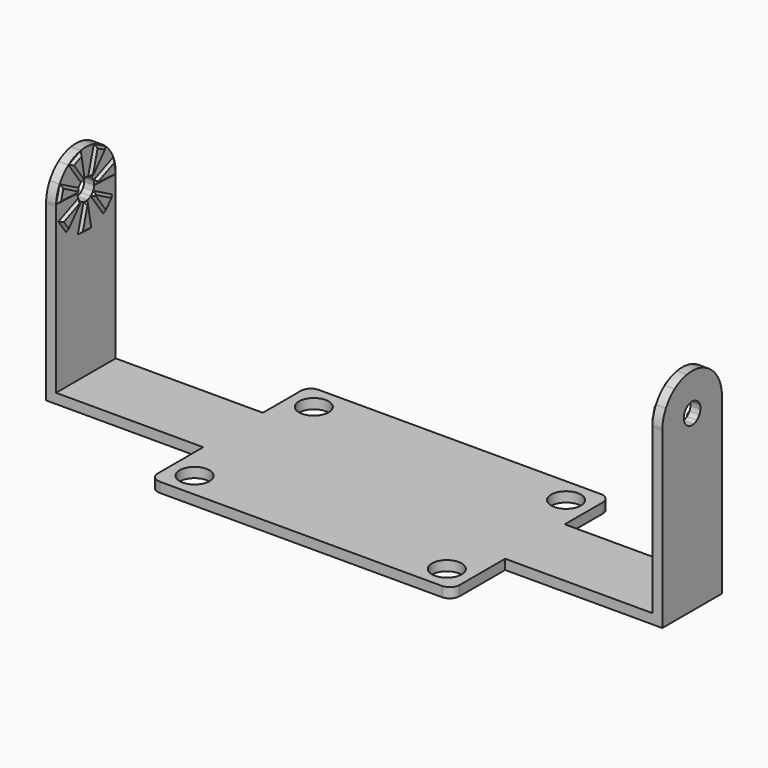
from build123d import *

# Parameters (mm, degrees)
F0_R                     = 3
F1_DEPTH                 = 2
F3_W                     = 29.6193578921
F3_H                     = 8.8474444038
F3_H_2                   = 6.1525555962
F4_DEPTH                 = 2
F6_DEPTH                 = 2
F7_DEPTH                 = 2
F8_DEPTH                 = 0.5
DRAFT_F8_DRAFTED_ANGLE   = 45
DRAFT_F8_2_DRAFTED_ANGLE = 45
DRAFT_F8_3_DRAFTED_ANGLE = 45
DRAFT_F8_4_DRAFTED_ANGLE = 45
DRAFT_F8_5_DRAFTED_ANGLE = 45
DRAFT_F8_6_DRAFTED_ANGLE = 45
DRAFT_F8_7_DRAFTED_ANGLE = 45


# Not quite as in the source:
# - an extrude with a draft is written as a straight extrude whose walls are then drafted
# - a feature names something its author has since deleted; it is built from what else it names


with BuildPart() as f1:
    # F0 (on Top) → F1 (new body)
    with BuildSketch(Plane.XY):
        with BuildLine():
            Line((0, 20.4223022205), (-28.3806421079, 20.4223022205))
            ThreePointArc((-28.3806421079, 20.4223022205), (-29.7948556703, 19.8365157828), (-30.3806421079, 18.4223022205))
            Line((-30.3806421079, 18.4223022205), (-30.3806421079, -17.5776977795))
            ThreePointArc((-30.3806421079, -17.5776977795), (-29.7948556703, -18.9919113419), (-28.3806421079, -19.5776977795))
            Line((-28.3806421079, -19.5776977795), (0, -19.5776977795))
            Line((0, -19.5776977795), (0, 20.4223022205))
        make_face()
        with Locations((-25.3806421079, -14.5776977795)):
            Circle(F0_R, mode=Mode.SUBTRACT)
        with Locations((-25.3806421079, 15.4223022205)):
            Circle(F0_R, mode=Mode.SUBTRACT)
    extrude(amount=F1_DEPTH)

    # F3 (on face) → F4 (join)
    with BuildSketch(Plane.XY.offset(2)):
        with Locations((-45.190321054, 4.4237222019)):
            Rectangle(F3_W, F3_H)
        with Locations((-45.190321054, -3.0762777981)):
            Rectangle(F3_W, F3_H_2)
    extrude(amount=-F4_DEPTH)

    # F5 (on face) → F6 (join)
    with BuildSketch(Plane(origin=(-60, 0, 0), x_dir=(0, -1, 0), z_dir=(-1, 0, 0))):
        with BuildLine():
            ThreePointArc((5.5633466733, 32.0864426173), (6.0037777081, 33.5139190004), (6.1525555962, 35.0003689528))
            ThreePointArc((6.1525555962, 35.0003689528), (6.1502334534, 35.1869882142), (6.1432684632, 35.373491914))
            Line((6.1432684632, 35.373491914), (5.5633466733, 32.0864426173))
        make_face()
        with BuildLine():
            Line((6.1525555962, 2), (6.1525555962, 35.0003689528))
            ThreePointArc((6.1525555962, 35.0003689528), (6.0037777081, 33.5139190004), (5.5633466733, 32.0864426173))
            ThreePointArc((5.5633466733, 32.0864426173), (4.7416691029, 30.6217051494), (3.6146579553, 29.3765321684))
            ThreePointArc((3.6146579553, 29.3765321684), (2.2388262755, 28.4133618467), (0.6831640089, 27.7804915664))
            ThreePointArc((0.6831640089, 27.7804915664), (-0.9743214426, 27.5096560858), (-2.6505168374, 27.6144362268))
            ThreePointArc((-2.6505168374, 27.6144362268), (-4.2613707393, 28.0895778756), (-5.7261082072, 28.9112554461))
            ThreePointArc((-5.7261082072, 28.9112554461), (-6.9712811882, 30.0382665936), (-7.9344515098, 31.4140982734))
            ThreePointArc((-7.9344515098, 31.4140982734), (-8.5673217902, 32.96976054), (-8.8381572708, 34.6272459916))
            ThreePointArc((-8.8381572708, 34.6272459916), (-8.8451176686, 34.8135652721), (-8.8474443948, 35))
            Line((-8.8474444038, 35), (-8.8474444038, 2))
            Line((-8.8474444038, 2), (6.1525555962, 2))
        make_face()
        with BuildLine():
            Line((5.2395627022, 38.5866396321), (6.1432684632, 35.373491914))
            ThreePointArc((6.1432684632, 35.373491914), (5.8724329825, 37.0309773655), (5.2395627022, 38.5866396321))
        make_face()
        with BuildLine():
            Line((0.7499551989, 35.1048433819), (6.1432684632, 35.373491914))
            Line((6.1432684632, 35.373491914), (5.2395627022, 38.5866396321))
            Line((5.2395627022, 38.5866396321), (0.4969175858, 36.004524743))
            ThreePointArc((0.4969175858, 36.004524743), (0.6741212644, 35.5689393083), (0.7499551989, 35.1048433819))
        make_face()
        with BuildLine():
            Line((5.5633466733, 32.0864426173), (6.1432684632, 35.373491914))
            Line((6.1432684632, 35.373491914), (0.7499551989, 35.1048433819))
            ThreePointArc((0.7499551989, 35.1048433819), (0.7519053962, 35.052622346), (0.7525555962, 35.0003689528))
            ThreePointArc((0.7525555962, 35.0003689528), (0.7108977875, 34.5841629661), (0.5875770978, 34.1844695788))
            Line((0.5875770978, 34.1844695788), (5.5633466733, 32.0864426173))
        make_face()
        with BuildLine():
            ThreePointArc((3.6146579553, 29.3765321684), (4.7416691029, 30.6217051494), (5.5633466733, 32.0864426173))
            Line((5.5633466733, 32.0864426173), (3.6146579553, 29.3765321684))
        make_face()
        with BuildLine():
            Line((3.6146579553, 29.3765321684), (5.5633466733, 32.0864426173))
            Line((5.5633466733, 32.0864426173), (0.5875770978, 34.1844695788))
            ThreePointArc((0.5875770978, 34.1844695788), (0.357507378, 33.7743430878), (0.0419442567, 33.4256946531))
            Line((0.0419442567, 33.4256946531), (3.6146579553, 29.3765321684))
        make_face()
        with BuildLine():
            Line((3.0312193995, 41.0894824594), (5.2395627022, 38.5866396321))
            ThreePointArc((5.2395627022, 38.5866396321), (4.2763923806, 39.9624713119), (3.0312193995, 41.0894824594))
        make_face()
        with BuildLine():
            Line((0.4969175858, 36.004524743), (5.2395627022, 38.5866396321))
            Line((5.2395627022, 38.5866396321), (3.0312193995, 41.0894824594))
            Line((3.0312193995, 41.0894824594), (-0.1214185389, 36.7053207346))
            ThreePointArc((-0.1214185389, 36.7053207346), (0.2272298958, 36.3897576133), (0.4969175858, 36.004524743))
        make_face()
        with BuildLine():
            ThreePointArc((0.6831640089, 27.7804915664), (2.2388262755, 28.4133618467), (3.6146579553, 29.3765321684))
            Line((3.6146579553, 29.3765321684), (0.6831640089, 27.7804915664))
        make_face()
        with BuildLine():
            Line((0.6831640089, 27.7804915664), (3.6146579553, 29.3765321684))
            Line((3.6146579553, 29.3765321684), (0.0419442567, 33.4256946531))
            ThreePointArc((0.0419442567, 33.4256946531), (-0.3432886136, 33.1560069631), (-0.7788740483, 32.9788032846))
            Line((-0.7788740483, 32.9788032846), (0.6831640089, 27.7804915664))
        make_face()
        with BuildLine():
            Line((-0.0443719702, 42.3863016787), (3.0312193995, 41.0894824594))
            ThreePointArc((3.0312193995, 41.0894824594), (1.5664819316, 41.9111600299), (-0.0443719702, 42.3863016787))
        make_face()
        with BuildLine():
            Line((-0.1214185389, 36.7053207346), (3.0312193995, 41.0894824594))
            Line((3.0312193995, 41.0894824594), (-0.0443719702, 42.3863016787))
            Line((-0.0443719702, 42.3863016787), (-0.9825841224, 37.068430116))
            ThreePointArc((-0.9825841224, 37.068430116), (-0.5315450299, 36.9353904543), (-0.1214185389, 36.7053207346))
        make_face()
        with BuildLine():
            ThreePointArc((-2.6505168374, 27.6144362268), (-0.9743214426, 27.5096560858), (0.6831640089, 27.7804915664))
            Line((0.6831640089, 27.7804915664), (-2.6505168374, 27.6144362268))
        make_face()
        with BuildLine():
            Line((-2.6505168374, 27.6144362268), (0.6831640089, 27.7804915664))
            Line((0.6831640089, 27.7804915664), (-0.7788740483, 32.9788032846))
            ThreePointArc((-0.7788740483, 32.9788032846), (-1.2429699747, 32.90296935), (-1.7123046852, 32.9323077895))
            Line((-1.7123046852, 32.9323077895), (-2.6505168374, 27.6144362268))
        make_face()
        with BuildLine():
            ThreePointArc((-8.258235481, 37.9142952882), (-8.6987030755, 36.4866380877), (-8.8474443948, 35))
            ThreePointArc((-8.8474443948, 35), (-8.8451176686, 34.8135652721), (-8.8381572708, 34.6272459916))
            Line((-8.8381572708, 34.6272459916), (-8.258235481, 37.9142952882))
        make_face()
        with BuildLine():
            Line((-3.3780528165, 42.2202463391), (-0.0443719702, 42.3863016787))
            ThreePointArc((-0.0443719702, 42.3863016787), (-1.720567365, 42.4910818198), (-3.3780528165, 42.2202463391))
        make_face()
        with BuildLine():
            Line((-0.9825841224, 37.068430116), (-0.0443719702, 42.3863016787))
            Line((-0.0443719702, 42.3863016787), (-3.3780528165, 42.2202463391))
            Line((-3.3780528165, 42.2202463391), (-1.9160147594, 37.0219346209))
            ThreePointArc((-1.9160147594, 37.0219346209), (-1.451918833, 37.0977685555), (-0.9825841224, 37.068430116))
        make_face()
        with BuildLine():
            Line((-8.258235481, 37.9142952882), (-3.2824659054, 35.8162683267))
            ThreePointArc((-3.2824659054, 35.8162683267), (-3.0523961857, 36.2263948177), (-2.7368330644, 36.5750432524))
            Line((-2.7368330644, 36.5750432524), (-6.309546763, 40.6242057372))
            Line((-6.309546763, 40.6242057372), (-8.258235481, 37.9142952882))
        make_face()
        with BuildLine():
            ThreePointArc((-3.4448440066, 34.8958945236), (-3.4155055671, 35.3652292342), (-3.2824659054, 35.8162683267))
            Line((-3.2824659054, 35.8162683267), (-8.258235481, 37.9142952882))
            Line((-8.258235481, 37.9142952882), (-8.8381572708, 34.6272459916))
            Line((-8.8381572708, 34.6272459916), (-3.4448440066, 34.8958945236))
        make_face()
        with BuildLine():
            Line((-6.309546763, 40.6242057372), (-2.7368330644, 36.5750432524))
            ThreePointArc((-2.7368330644, 36.5750432524), (-2.351600194, 36.8447309424), (-1.9160147594, 37.0219346209))
            Line((-1.9160147594, 37.0219346209), (-3.3780528165, 42.2202463391))
            Line((-3.3780528165, 42.2202463391), (-6.309546763, 40.6242057372))
        make_face()
        with BuildLine():
            Line((-2.6505168374, 27.6144362268), (-1.7123046852, 32.9323077895))
            ThreePointArc((-1.7123046852, 32.9323077895), (-2.1633437778, 33.0653474512), (-2.5734702688, 33.2954171709))
            Line((-2.5734702688, 33.2954171709), (-5.7261082072, 28.9112554461))
            Line((-5.7261082072, 28.9112554461), (-2.6505168374, 27.6144362268))
        make_face()
        with BuildLine():
            Line((-5.7261082072, 28.9112554461), (-2.5734702688, 33.2954171709))
            ThreePointArc((-2.5734702688, 33.2954171709), (-2.9221187035, 33.6109802922), (-3.1918063935, 33.9962131625))
            Line((-3.1918063935, 33.9962131625), (-7.9344515098, 31.4140982734))
            Line((-7.9344515098, 31.4140982734), (-5.7261082072, 28.9112554461))
        make_face()
        with BuildLine():
            Line((-7.9344515098, 31.4140982734), (-3.1918063935, 33.9962131625))
            ThreePointArc((-3.1918063935, 33.9962131625), (-3.369010072, 34.4317985972), (-3.4448440066, 34.8958945236))
            Line((-3.4448440066, 34.8958945236), (-8.8381572708, 34.6272459916))
            Line((-8.8381572708, 34.6272459916), (-7.9344515098, 31.4140982734))
        make_face()
        with BuildLine():
            ThreePointArc((-5.7261082072, 28.9112554461), (-4.2613707393, 28.0895778756), (-2.6505168374, 27.6144362268))
            Line((-2.6505168374, 27.6144362268), (-5.7261082072, 28.9112554461))
        make_face()
        with BuildLine():
            ThreePointArc((-6.309546763, 40.6242057372), (-7.4365579105, 39.3790327561), (-8.258235481, 37.9142952882))
            Line((-8.258235481, 37.9142952882), (-6.309546763, 40.6242057372))
        make_face()
        with BuildLine():
            Line((-7.9344515098, 31.4140982734), (-8.8381572708, 34.6272459916))
            ThreePointArc((-8.8381572708, 34.6272459916), (-8.5673217902, 32.96976054), (-7.9344515098, 31.4140982734))
        make_face()
        with BuildLine():
            Line((-6.309546763, 40.6242057372), (-3.3780528165, 42.2202463391))
            ThreePointArc((-3.3780528165, 42.2202463391), (-4.9337150832, 41.5873760588), (-6.309546763, 40.6242057372))
        make_face()
        with BuildLine():
            ThreePointArc((-7.9344515098, 31.4140982734), (-6.9712811882, 30.0382665936), (-5.7261082072, 28.9112554461))
            Line((-5.7261082072, 28.9112554461), (-7.9344515098, 31.4140982734))
        make_face()
    extrude(amount=F6_DEPTH)

    # F7 (add): a face of the model
    f7_faces = [f1.faces().sort_by_distance(p)[0] for p in [
        (-60, 1.3474444038, 1),
    ]]
    extrude(f7_faces, amount=F7_DEPTH)


with BuildPart() as f8_drafted:
    # F5 (on face) → F8 (new body)
    with BuildSketch(Plane(origin=(-60, 0, 0), x_dir=(0, -1, 0), z_dir=(-1, 0, 0))):
        with BuildLine():
            Line((3.6146579553, 29.3765321684), (5.5633466733, 32.0864426173))
            Line((5.5633466733, 32.0864426173), (0.5875770978, 34.1844695788))
            ThreePointArc((0.5875770978, 34.1844695788), (0.357507378, 33.7743430878), (0.0419442567, 33.4256946531))
            Line((0.0419442567, 33.4256946531), (3.6146579553, 29.3765321684))
        make_face()
    extrude(amount=-F8_DEPTH)

    # draft_F8_drafted
    draft_f8_drafted_walls = [f8_drafted.faces().sort_by_distance(p)[0] for p in [
        (-59.6666666667, -0.357507378, 33.7743430878),
        (-59.6666666667, -1.828301106, 31.4011134107),
        (-59.6666666667, -4.5890023143, 30.7314873928),
        (-59.6666666667, -3.0754618855, 33.1354560981),
    ]]
    draft(draft_f8_drafted_walls, neutral_plane=Plane(origin=(-60, 0, 0), x_dir=(0, -1, 0), z_dir=(1, 0, 0)), angle=DRAFT_F8_DRAFTED_ANGLE)


with BuildPart() as f1_1:
    add(f1.part)

    # join_F8_drafted: union F8_drafted
    add(f8_drafted.part)


with BuildPart() as f8_2_drafted:
    # F5 (on face) → F8, piece 2 (new body)
    with BuildSketch(Plane(origin=(-60, 0, 0), x_dir=(0, -1, 0), z_dir=(-1, 0, 0))):
        with BuildLine():
            Line((0.7499551989, 35.1048433819), (6.1432684632, 35.373491914))
            Line((6.1432684632, 35.373491914), (5.2395627022, 38.5866396321))
            Line((5.2395627022, 38.5866396321), (0.4969175858, 36.004524743))
            ThreePointArc((0.4969175858, 36.004524743), (0.6741212644, 35.5689393083), (0.7499551989, 35.1048433819))
        make_face()
    extrude(amount=-F8_DEPTH)

    # draft_F8_2_drafted
    draft_f8_2_drafted_walls = [f8_2_drafted.faces().sort_by_distance(p)[0] for p in [
        (-59.6666666667, -0.6741212644, 35.5689393083),
        (-59.6666666667, -3.446611831, 35.2391676479),
        (-59.6666666667, -5.6914155827, 36.980065773),
        (-59.6666666667, -2.868240144, 37.2955821875),
    ]]
    draft(draft_f8_2_drafted_walls, neutral_plane=Plane(origin=(-60, 0, 0), x_dir=(0, -1, 0), z_dir=(1, 0, 0)), angle=DRAFT_F8_2_DRAFTED_ANGLE)


with BuildPart() as f1_2:
    add(f1_1.part)

    # join_F8_2_drafted: union F8_2_drafted
    add(f8_2_drafted.part)


with BuildPart() as f8_3_drafted:
    # F5 (on face) → F8, piece 3 (new body)
    with BuildSketch(Plane(origin=(-60, 0, 0), x_dir=(0, -1, 0), z_dir=(-1, 0, 0))):
        with BuildLine():
            Line((-0.1214185389, 36.7053207346), (3.0312193995, 41.0894824594))
            Line((3.0312193995, 41.0894824594), (-0.0443719702, 42.3863016787))
            Line((-0.0443719702, 42.3863016787), (-0.9825841224, 37.068430116))
            ThreePointArc((-0.9825841224, 37.068430116), (-0.5315450299, 36.9353904543), (-0.1214185389, 36.7053207346))
        make_face()
    extrude(amount=-F8_DEPTH)

    # draft_F8_3_drafted
    draft_f8_3_drafted_walls = [f8_3_drafted.faces().sort_by_distance(p)[0] for p in [
        (-59.6666666667, -1.4549004303, 38.897401597),
        (-59.6666666667, -1.4934237146, 41.7378920691),
        (-59.6666666667, 0.5134780463, 39.7273658974),
        (-59.6666666667, 0.5315450299, 36.9353904543),
    ]]
    draft(draft_f8_3_drafted_walls, neutral_plane=Plane(origin=(-60, 0, 0), x_dir=(0, -1, 0), z_dir=(1, 0, 0)), angle=DRAFT_F8_3_DRAFTED_ANGLE)


with BuildPart() as f1_3:
    add(f1_2.part)

    # join_F8_3_drafted: union F8_3_drafted
    add(f8_3_drafted.part)


with BuildPart() as f8_4_drafted:
    # F5 (on face) → F8, piece 4 (new body)
    with BuildSketch(Plane(origin=(-60, 0, 0), x_dir=(0, -1, 0), z_dir=(-1, 0, 0))):
        with BuildLine():
            Line((-6.309546763, 40.6242057372), (-2.7368330644, 36.5750432524))
            ThreePointArc((-2.7368330644, 36.5750432524), (-2.351600194, 36.8447309424), (-1.9160147594, 37.0219346209))
            Line((-1.9160147594, 37.0219346209), (-3.3780528165, 42.2202463391))
            Line((-3.3780528165, 42.2202463391), (-6.309546763, 40.6242057372))
        make_face()
    extrude(amount=-F8_DEPTH)

    # draft_F8_4_drafted
    draft_f8_4_drafted_walls = [f8_4_drafted.faces().sort_by_distance(p)[0] for p in [
        (-59.6666666667, 2.647033788, 39.62109048),
        (-59.6666666667, 4.8437997898, 41.4222260381),
        (-59.6666666667, 4.5231899137, 38.5996244948),
        (-59.6666666667, 2.351600194, 36.8447309424),
    ]]
    draft(draft_f8_4_drafted_walls, neutral_plane=Plane(origin=(-60, 0, 0), x_dir=(0, -1, 0), z_dir=(1, 0, 0)), angle=DRAFT_F8_4_DRAFTED_ANGLE)


with BuildPart() as f1_4:
    add(f1_3.part)

    # join_F8_4_drafted: union F8_4_drafted
    add(f8_4_drafted.part)


with BuildPart() as f8_5_drafted:
    # F5 (on face) → F8, piece 5 (new body)
    with BuildSketch(Plane(origin=(-60, 0, 0), x_dir=(0, -1, 0), z_dir=(-1, 0, 0))):
        with BuildLine():
            ThreePointArc((-3.4448440066, 34.8958945236), (-3.4155055671, 35.3652292342), (-3.2824659054, 35.8162683267))
            Line((-3.2824659054, 35.8162683267), (-8.258235481, 37.9142952882))
            Line((-8.258235481, 37.9142952882), (-8.8381572708, 34.6272459916))
            Line((-8.8381572708, 34.6272459916), (-3.4448440066, 34.8958945236))
        make_face()
    extrude(amount=-F8_DEPTH)

    # draft_F8_5_drafted
    draft_f8_5_drafted_walls = [f8_5_drafted.faces().sort_by_distance(p)[0] for p in [
        (-59.6666666667, 5.7703506932, 36.8652818074),
        (-59.6666666667, 8.5481963759, 36.2707706399),
        (-59.6666666667, 6.1415006387, 34.7615702576),
        (-59.6666666667, 3.4155055671, 35.3652292342),
    ]]
    draft(draft_f8_5_drafted_walls, neutral_plane=Plane(origin=(-60, 0, 0), x_dir=(0, -1, 0), z_dir=(1, 0, 0)), angle=DRAFT_F8_5_DRAFTED_ANGLE)


with BuildPart() as f1_5:
    add(f1_4.part)

    # join_F8_5_drafted: union F8_5_drafted
    add(f8_5_drafted.part)


with BuildPart() as f8_6_drafted:
    # F5 (on face) → F8, piece 6 (new body)
    with BuildSketch(Plane(origin=(-60, 0, 0), x_dir=(0, -1, 0), z_dir=(-1, 0, 0))):
        with BuildLine():
            Line((-5.7261082072, 28.9112554461), (-2.5734702688, 33.2954171709))
            ThreePointArc((-2.5734702688, 33.2954171709), (-2.9221187035, 33.6109802922), (-3.1918063935, 33.9962131625))
            Line((-3.1918063935, 33.9962131625), (-7.9344515098, 31.4140982734))
            Line((-7.9344515098, 31.4140982734), (-5.7261082072, 28.9112554461))
        make_face()
    extrude(amount=-F8_DEPTH)

    # draft_F8_6_drafted
    draft_f8_6_drafted_walls = [f8_6_drafted.faces().sort_by_distance(p)[0] for p in [
        (-59.6666666667, 5.5631289517, 32.705155718),
        (-59.6666666667, 6.8302798585, 30.1626768597),
        (-59.6666666667, 4.149789238, 31.1033363085),
        (-59.6666666667, 2.9221187035, 33.6109802922),
    ]]
    draft(draft_f8_6_drafted_walls, neutral_plane=Plane(origin=(-60, 0, 0), x_dir=(0, -1, 0), z_dir=(1, 0, 0)), angle=DRAFT_F8_6_DRAFTED_ANGLE)


with BuildPart() as f1_6:
    add(f1_5.part)

    # join_F8_6_drafted: union F8_6_drafted
    add(f8_6_drafted.part)


with BuildPart() as f8_7_drafted:
    # F5 (on face) → F8, piece 7 (new body)
    with BuildSketch(Plane(origin=(-60, 0, 0), x_dir=(0, -1, 0), z_dir=(-1, 0, 0))):
        with BuildLine():
            Line((-2.6505168374, 27.6144362268), (0.6831640089, 27.7804915664))
            Line((0.6831640089, 27.7804915664), (-0.7788740483, 32.9788032846))
            ThreePointArc((-0.7788740483, 32.9788032846), (-1.2429699747, 32.90296935), (-1.7123046852, 32.9323077895))
            Line((-1.7123046852, 32.9323077895), (-2.6505168374, 27.6144362268))
        make_face()
    extrude(amount=-F8_DEPTH)

    # draft_F8_7_drafted
    draft_f8_7_drafted_walls = [f8_7_drafted.faces().sort_by_distance(p)[0] for p in [
        (-59.6666666667, 1.2429699747, 32.90296935),
        (-59.6666666667, 2.1814107613, 30.2733720081),
        (-59.6666666667, 0.9836764143, 27.6974638966),
        (-59.6666666667, 0.0478550197, 30.3796474255),
    ]]
    draft(draft_f8_7_drafted_walls, neutral_plane=Plane(origin=(-60, 0, 0), x_dir=(0, -1, 0), z_dir=(1, 0, 0)), angle=DRAFT_F8_7_DRAFTED_ANGLE)


with BuildPart() as f1_7:
    add(f1_6.part)

    # join_F8_7_drafted: union F8_7_drafted
    add(f8_7_drafted.part)

    # F9: F1 across plane


with BuildPart() as f1_8:
    add(f1_7.part)
    add(f1_7.part.mirror(Plane.YZ))


solid = f1_8.part
